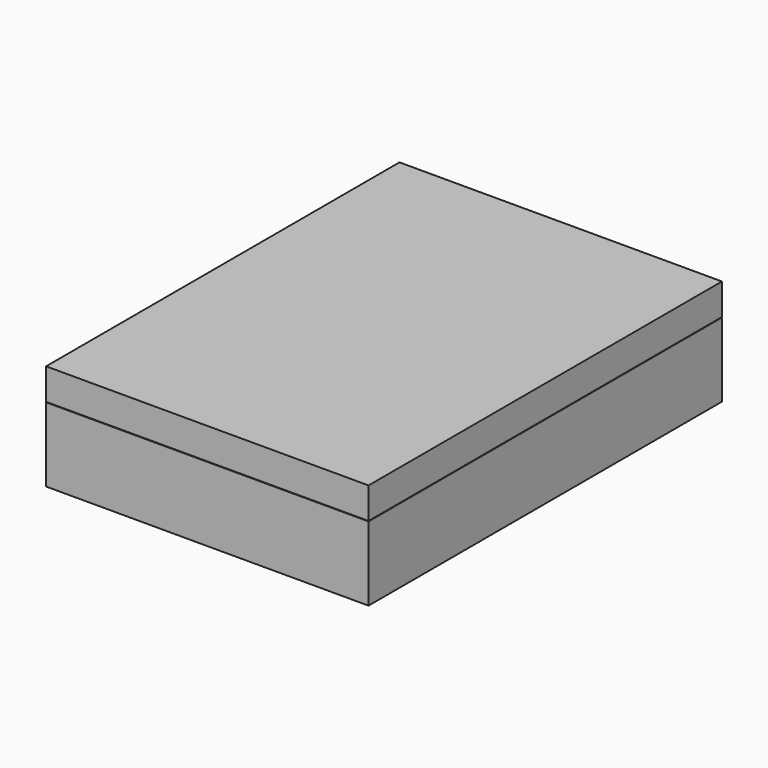
from build123d import *

# Parameters (mm, degrees)
F3_W      = 72.2
F3_H      = 98.9
F4_DEPTH  = 1
F5_W      = 72.2
F5_H      = 98.9
F5_W_2    = 65.2
F5_H_2    = 91.9
F6_DEPTH  = 21.6
F8_W      = 72.2
F8_H      = 98.9
F8_W_2    = 68.4
F8_H_2    = 95.1
F9_DEPTH  = 6
F10_W     = 72.2
F10_H     = 98.9
F11_DEPTH = 1
F12_W     = 72.2
F12_H     = 98.9
F12_W_2   = 69
F12_H_2   = 95.7
F13_DEPTH = 6


with BuildPart() as f4:
    # F3 (on Top) → F4 (new body)
    with BuildSketch(Plane.XY):
        Rectangle(F3_W, F3_H)
    extrude(amount=F4_DEPTH)

    # F5 (on face) → F6 (join)
    with BuildSketch(Plane.XY.offset(1)):
        Rectangle(F5_W, F5_H)
        Rectangle(F5_W_2, F5_H_2, mode=Mode.SUBTRACT)
    extrude(amount=F6_DEPTH)

    # F8 (on face) → F9 (cut)
    with BuildSketch(Plane.XY.offset(22.6)):
        Rectangle(F8_W, F8_H)
        Rectangle(F8_W_2, F8_H_2, mode=Mode.SUBTRACT)
    extrude(amount=-F9_DEPTH, mode=Mode.SUBTRACT)


with BuildPart() as f11:
    # F10 (on face) → F11 (new body)
    with BuildSketch(Plane.XY.offset(22.7)):
        Rectangle(F10_W, F10_H)
    extrude(amount=F11_DEPTH)

    # F12 (on face) → F13 (join)
    with BuildSketch(Plane(origin=(0, 0, 22.7), x_dir=(1, 0, 0), z_dir=(0, 0, -1))):
        Rectangle(F12_W, F12_H)
        Rectangle(F12_W_2, F12_H_2, mode=Mode.SUBTRACT)
    extrude(amount=F13_DEPTH)


solid = Compound([f4.part, f11.part])
